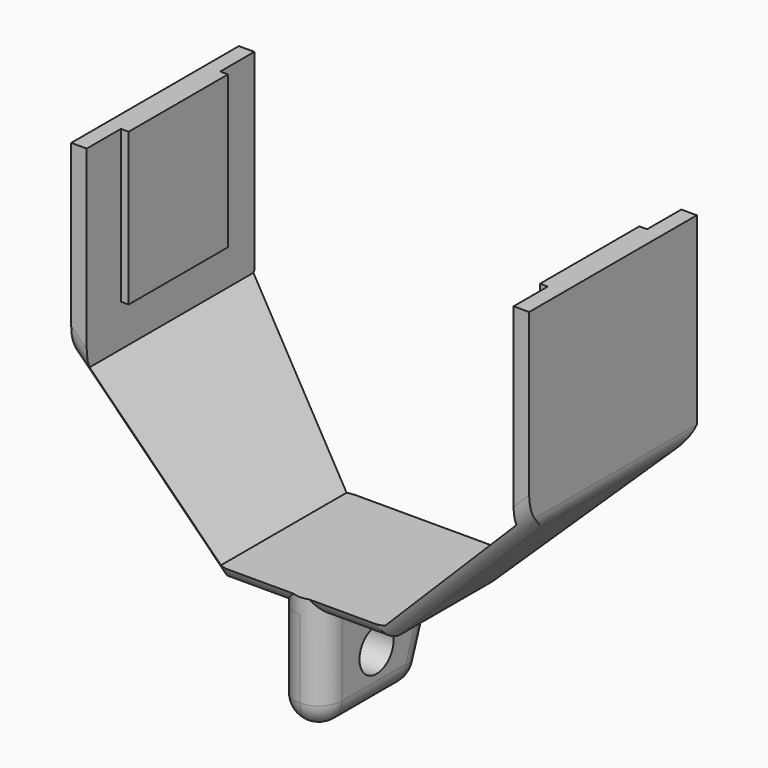
from build123d import *

# Parameters (mm, degrees)
F0_W          = 3
F0_H          = 13
F1_DEPTH      = 13.5
F2_W          = 16
F2_H          = 19.6
F3_DEPTH      = 1
F6_DEPTH      = 5000
F7_R          = 2.75
F8_DEPTH      = 50
F9_F1_R       = 3
F9_F2_R       = 3
F9_F3_R       = 3
F9_F4_R       = 2.9999
F10_T1_DEPTH  = 15.0673355609
F10_T3_DEPTH  = 15.0673355609
F10_T5_DEPTH  = 41.7748308216
F10_T7_DEPTH  = 41.7748308216
F10_T9_DEPTH  = 43.4696886285
F10_T11_DEPTH = 12.8188920975
F10_T13_DEPTH = 12.8188920975
F10_T15_DEPTH = 43.4696886285
F10_T17_DEPTH = 33.2132034356
F10_T22_DEPTH = 8.2514565366
F10_S23_R     = 3
F10_T24_DEPTH = 6
F10_T28_DEPTH = 8.2515565366
F10_S29_R     = 3
F10_T30_DEPTH = 6
F10_T34_DEPTH = 10.4999
F10_S35_R     = 3
F10_T36_DEPTH = 7
F10_T40_DEPTH = 10.5
F10_S41_R     = 3
F10_T42_DEPTH = 7


# Not quite as in the source:
# - a fillet or chamfer that OpenCascade refuses, or shapes differently, is made with other operations: its cross-section is extruded or revolved along the edge and cut away or added
# - a fillet or chamfer is up to 0.001 mm smaller than in the source, because OpenCascade refuses the exact size
# - a feature names something its author has since deleted; it is built from what else it names


with BuildPart() as f1:
    # F0 (on Front) → F1 (new body, symmetric)
    with BuildSketch(Plane.XZ):
        with Locations((-1.5, -25.4326644391)):
            Rectangle(F0_W, F0_H)
        Polygon((-10.5673355609, -16.9326644391), (-27.5, 0), (-27.5, 3.3434056677), (-27.5, 25), (-29.5, 25), (-29.5, 0), (-10.5673355609, -18.9326644391), (-3, -18.9326644391), (0, -18.9326644391), (0, -16.9326644391), align=None)
    extrude(amount=F1_DEPTH, both=True)

    # F2 (on face) → F3 (join)
    with BuildSketch(Plane.YZ.offset(-27.5)):
        with Locations((0, 15.2)):
            Rectangle(F2_W, F2_H)
    extrude(amount=F3_DEPTH)

    # F4: F1 across plane


with BuildPart() as f1_1:
    add(f1.part)
    add(f1.part.mirror(Plane.YZ))

    # F5 (on face) → F6 (cut, symmetric)
    with BuildSketch(Plane(origin=(-29.5, 0, 0), x_dir=(0, -1, 0), z_dir=(-1, 0, 0))):
        Polygon((-13.5, 0), (-21.2256871164, 0), (-25.0640398382, -39.3923101205), (-6.5540728933, -39.3923101205), (0.180805733, -37.5877048314), align=None)
    extrude(amount=F6_DEPTH, both=True, mode=Mode.SUBTRACT)

    # F7 (on face) → F8 (cut, symmetric)
    with BuildSketch(Plane.YZ.offset(3)):
        with Locations((-4.9499999732, -25.3868680447)):
            Circle(F7_R)
    extrude(amount=F8_DEPTH, both=True, mode=Mode.SUBTRACT)

    # F9: fillet of radius 3 on 4 edges, made by hand

    # F9_f1
    f9_f1_edges = [f1_1.edges().sort_by_distance(p)[0] for p in [
        (0, 1.8774606434, -31.9326644391),
    ]]
    fillet(f9_f1_edges, radius=F9_F1_R)

    # F9_f2
    f9_f2_edges = [f1_1.edges().sort_by_distance(p)[0] for p in [
        (0, -13.5, -31.9326644391),
    ]]
    fillet(f9_f2_edges, radius=F9_F2_R)

    # F9_f3
    f9_f3_edges = [f1_1.edges().sort_by_distance(p)[0] for p in [
        (3, -5.3615809856, -31.9326644391),
    ]]
    fillet(f9_f3_edges, radius=F9_F3_R)

    # F9_f4 (radius 3 in the source; OpenCascade refuses exactly that, so slightly less here)
    f9_f4_edges = [f1_1.edges().sort_by_distance(p)[0] for p in [
        (-3, -5.3615809856, -31.9326644391),
    ]]
    fillet(f9_f4_edges, radius=F9_F4_R)

    # F10: fillet of radius 3 on 12 edges, made by hand

    # F10_s2 → F10_t1 (cut)
    with BuildSketch(Plane.YZ.offset(3)):
        with BuildLine():
            ThreePointArc((-13.5, -15.9326644391), (-12.6213203436, -18.0539847826), (-10.5, -18.9326644391))
            Line((-10.5, -18.9326644391), (-13.5, -18.9326644391))
            Line((-13.5, -18.9326644391), (-13.5, -15.9326644391))
        make_face()
    extrude(amount=F10_T1_DEPTH, mode=Mode.SUBTRACT)

    # F10_s4 → F10_t3 (cut)
    with BuildSketch(Plane.YZ.offset(-18.0673355609)):
        with BuildLine():
            ThreePointArc((-13.5, -15.9326644391), (-12.6213203436, -18.0539847826), (-10.5, -18.9326644391))
            Line((-10.5, -18.9326644391), (-13.5, -18.9326644391))
            Line((-13.5, -18.9326644391), (-13.5, -15.9326644391))
        make_face()
    extrude(amount=F10_T3_DEPTH, mode=Mode.SUBTRACT)

    # F10_s6 → F10_t5 (cut)
    with BuildSketch(Plane(origin=(-20.0533008589, 0, 20.0533008589), x_dir=(0, 1, 0), z_dir=(0.7071067812, 0, -0.7071067812))):
        with BuildLine():
            ThreePointArc((-13.5, -17.859650045), (-12.6213203436, -19.9809703886), (-10.5, -20.859650045))
            Line((-10.5, -20.859650045), (-13.5, -20.859650045))
            Line((-13.5, -20.859650045), (-13.5, -17.859650045))
        make_face()
    extrude(amount=F10_T5_DEPTH, mode=Mode.SUBTRACT)

    # F10_s8 → F10_t7 (cut)
    with BuildSketch(Plane(origin=(20.0533008589, 0, 20.0533008589), x_dir=(0, 1, 0), z_dir=(-0.7071067812, 0, -0.7071067812))):
        with BuildLine():
            ThreePointArc((-13.5, 17.859650045), (-12.6213203436, 19.9809703886), (-10.5, 20.859650045))
            Line((-10.5, 20.859650045), (-13.5, 20.859650045))
            Line((-13.5, 20.859650045), (-13.5, 17.859650045))
        make_face()
    extrude(amount=F10_T7_DEPTH, mode=Mode.SUBTRACT)

    # F10_s10 → F10_t9 (cut)
    with BuildSketch(Plane(origin=(-6.8077517267, -2.4778189908, -6.8077517267), x_dir=(-0.3420201433, 0.9396926208, 0), z_dir=(0.6847910788, 0.2492435694, 0.6847910788))):
        with BuildLine():
            ThreePointArc((0.3217904404, -21.5780178201), (2.267861443, -21.4075638122), (3.6963913931, -20.0750664959))
            Line((3.6963913931, -20.0750664959), (2.5962561525, -22.1449137726))
            Line((2.5962561525, -22.1449137726), (0.3217904404, -21.5780178201))
        make_face()
    extrude(amount=F10_T9_DEPTH, mode=Mode.SUBTRACT)

    # F10_s12 → F10_t11 (cut)
    with BuildSketch(Plane.YZ.offset(3)):
        with BuildLine():
            ThreePointArc((4.5084510742, -18.9326644391), (6.2291803832, -18.3901205719), (7.3275289366, -16.9587248691))
            Line((7.3275289366, -16.9587248691), (6.6090736888, -18.9326644391))
            Line((6.6090736888, -18.9326644391), (4.5084510742, -18.9326644391))
        make_face()
    extrude(amount=F10_T11_DEPTH, mode=Mode.SUBTRACT)

    # F10_s14 → F10_t13 (cut)
    with BuildSketch(Plane.YZ.offset(-15.8188920975)):
        with BuildLine():
            ThreePointArc((4.5084510742, -18.9326644391), (6.2291803832, -18.3901205719), (7.3275289366, -16.9587248691))
            Line((7.3275289366, -16.9587248691), (6.6090736888, -18.9326644391))
            Line((6.6090736888, -18.9326644391), (4.5084510742, -18.9326644391))
        make_face()
    extrude(amount=F10_T13_DEPTH, mode=Mode.SUBTRACT)

    # F10_s16 → F10_t15 (cut)
    with BuildSketch(Plane(origin=(6.8077517267, -2.4778189908, -6.8077517267), x_dir=(-0.3420201433, -0.9396926208, 0), z_dir=(-0.6847910788, 0.2492435694, 0.6847910788))):
        with BuildLine():
            ThreePointArc((-0.3217904404, -21.5780178201), (-2.267861443, -21.4075638122), (-3.6963913931, -20.0750664959))
            Line((-3.6963913931, -20.0750664959), (-2.5962561525, -22.1449137726))
            Line((-2.5962561525, -22.1449137726), (-0.3217904404, -21.5780178201))
        make_face()
    extrude(amount=F10_T15_DEPTH, mode=Mode.SUBTRACT)

    # F10_s18 → F10_t17 (cut)
    with BuildSketch(Plane.XZ.offset(-16.6066017178)):
        with BuildLine():
            ThreePointArc((28.6213203436, -0.8786796564), (29.2716385975, 0.09459039), (29.5, 1.2426406871))
            Line((29.5, 1.2426406871), (29.5, 0))
            Line((29.5, 0), (28.6213203436, -0.8786796564))
        make_face()
        with BuildLine():
            ThreePointArc((-28.6213203436, -0.8786796564), (-29.2716385975, 0.09459039), (-29.5, 1.2426406871))
            Line((-29.5, 1.2426406871), (-29.5, 0))
            Line((-29.5, 0), (-28.6213203436, -0.8786796564))
        make_face()
    extrude(amount=F10_T17_DEPTH, mode=Mode.SUBTRACT)


with BuildPart() as f10_tool20:
    # F10_s21 → F10_t22 (new body)
    with BuildSketch(Plane.YZ.offset(-3)):
        with BuildLine():
            ThreePointArc((4.5084510742, -18.9326644391), (6.2291803832, -18.3901205719), (7.3275289366, -16.9587248691))
            Line((7.3275289366, -16.9587248691), (6.6090736888, -18.9326644391))
            Line((6.6090736888, -18.9326644391), (4.5084510742, -18.9326644391))
        make_face()
    extrude(amount=F10_T22_DEPTH)

    # F10_s23 → F10_t24 (cut, symmetric)
    with BuildSketch(Plane(origin=(0, -5.0618981212, -13.9074507876), x_dir=(1, 0, 0), z_dir=(0, 0.3420201433, 0.9396926208))):
        with Locations((0, 9.6858503806)):
            Circle(F10_S23_R)
    extrude(amount=F10_T24_DEPTH, both=True, mode=Mode.SUBTRACT)


with BuildPart() as f1_2:
    add(f1_1.part)

    # F10_t19: cut F10_tool20
    add(f10_tool20.part, mode=Mode.SUBTRACT)


with BuildPart() as f10_tool26:
    # F10_s27 → F10_t28 (new body)
    with BuildSketch(Plane.YZ.offset(3)):
        with BuildLine():
            ThreePointArc((4.5084510742, -18.9326644391), (6.2291803832, -18.3901205719), (7.3275289366, -16.9587248691))
            Line((7.3275289366, -16.9587248691), (6.6090736888, -18.9326644391))
            Line((6.6090736888, -18.9326644391), (4.5084510742, -18.9326644391))
        make_face()
    extrude(amount=-F10_T28_DEPTH)

    # F10_s29 → F10_t30 (cut, symmetric)
    with BuildSketch(Plane(origin=(0, -5.0618981212, -13.9074507876), x_dir=(1, 0, 0), z_dir=(0, 0.3420201433, 0.9396926208))):
        with Locations((0, 9.6858503806)):
            Circle(F10_S29_R)
    extrude(amount=F10_T30_DEPTH, both=True, mode=Mode.SUBTRACT)


with BuildPart() as f1_3:
    add(f1_2.part)

    # F10_t25: cut F10_tool26
    add(f10_tool26.part, mode=Mode.SUBTRACT)


with BuildPart() as f10_tool32:
    # F10_s33 → F10_t34 (new body)
    with BuildSketch(Plane.YZ.offset(-3)):
        with BuildLine():
            ThreePointArc((-13.5, -15.9326644391), (-12.6213203436, -18.0539847826), (-10.5, -18.9326644391))
            Line((-10.5, -18.9326644391), (-13.5, -18.9326644391))
            Line((-13.5, -18.9326644391), (-13.5, -15.9326644391))
        make_face()
    extrude(amount=F10_T34_DEPTH)

    # F10_s35 → F10_t36 (cut, symmetric)
    with BuildSketch(Plane.XY.offset(-17.4)):
        with Locations((0, -10.5)):
            Circle(F10_S35_R)
    extrude(amount=F10_T36_DEPTH, both=True, mode=Mode.SUBTRACT)


with BuildPart() as f1_4:
    add(f1_3.part)

    # F10_t31: cut F10_tool32
    add(f10_tool32.part, mode=Mode.SUBTRACT)


with BuildPart() as f10_tool38:
    # F10_s39 → F10_t40 (new body)
    with BuildSketch(Plane.YZ.offset(3)):
        with BuildLine():
            ThreePointArc((-13.5, -15.9326644391), (-12.6213203436, -18.0539847826), (-10.5, -18.9326644391))
            Line((-10.5, -18.9326644391), (-13.5, -18.9326644391))
            Line((-13.5, -18.9326644391), (-13.5, -15.9326644391))
        make_face()
    extrude(amount=-F10_T40_DEPTH)

    # F10_s41 → F10_t42 (cut, symmetric)
    with BuildSketch(Plane.XY.offset(-17.4)):
        with Locations((0, -10.5)):
            Circle(F10_S41_R)
    extrude(amount=F10_T42_DEPTH, both=True, mode=Mode.SUBTRACT)


with BuildPart() as f1_5:
    add(f1_4.part)

    # F10_t37: cut F10_tool38
    add(f10_tool38.part, mode=Mode.SUBTRACT)


solid = f1_5.part
